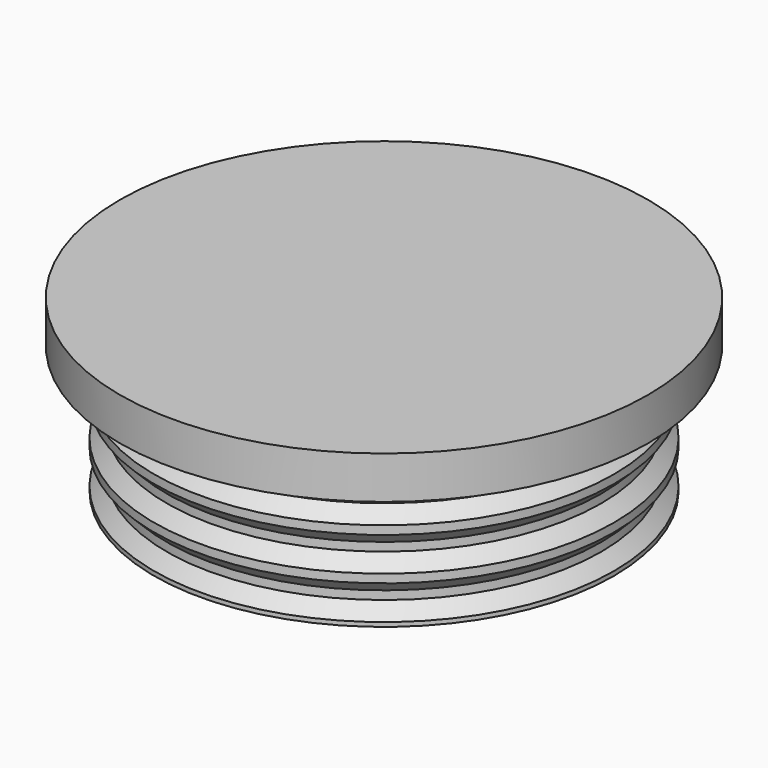
from build123d import *

# Parameters (mm, degrees)
F0_R     = 27
F0_R_2   = 22
F1_DEPTH = 15
F2_R     = 31
F2_R_2   = 27
F2_R_3   = 22
F3_DEPTH = 5
F4_W     = 1.5
F4_H     = 1
F6_SIZE2 = 1.49999
F6_SIZE  = 1.49999


# Not quite as in the source:
# - a fillet or chamfer is up to 0.001 mm smaller than in the source, because OpenCascade refuses the exact size


with BuildPart() as f1:
    # F0 (on Top) → F1 (new body)
    with BuildSketch(Plane.XY):
        Circle(F0_R)
        Circle(F0_R_2, mode=Mode.SUBTRACT)
    extrude(amount=F1_DEPTH)

    # F2 (on face) → F3 (join)
    with BuildSketch(Plane.XY.offset(15)):
        Circle(F2_R)
        Circle(F2_R_2, mode=Mode.SUBTRACT)
        Circle(F2_R_2)
        Circle(F2_R_3, mode=Mode.SUBTRACT)
        Circle(F2_R_3)
    extrude(amount=F3_DEPTH)

    # F4 (on Front) → F5 (revolve, cut)
    with BuildSketch(Plane.XZ):
        with Locations((-26.25, 2.5)):
            Rectangle(F4_W, F4_H)
        with Locations((-26.25, 7.5)):
            Rectangle(F4_W, F4_H)
        with Locations((-26.25, 12.5)):
            Rectangle(F4_W, F4_H)
    revolve(axis=Axis((0, 0, 9.1704530641), (0, 0, -1)), mode=Mode.SUBTRACT)

    # F6 (size 1.5 and 1.5 in the source; OpenCascade refuses exactly that, so slightly less here)
    f6_edges = [f1.edges().sort_by_distance(p)[0] for p in [
        (-27, 0, 3),
        (27, 0, 5),
        (-27, 0, 7),
        (-27, 0, 2),
        (-27, 0, 8),
        (27, 0, 10),
        (-27, 0, 12),
        (-27, 0, 13),
    ]]
    chamfer(f6_edges, length=F6_SIZE, length2=F6_SIZE2)


solid = f1.part
